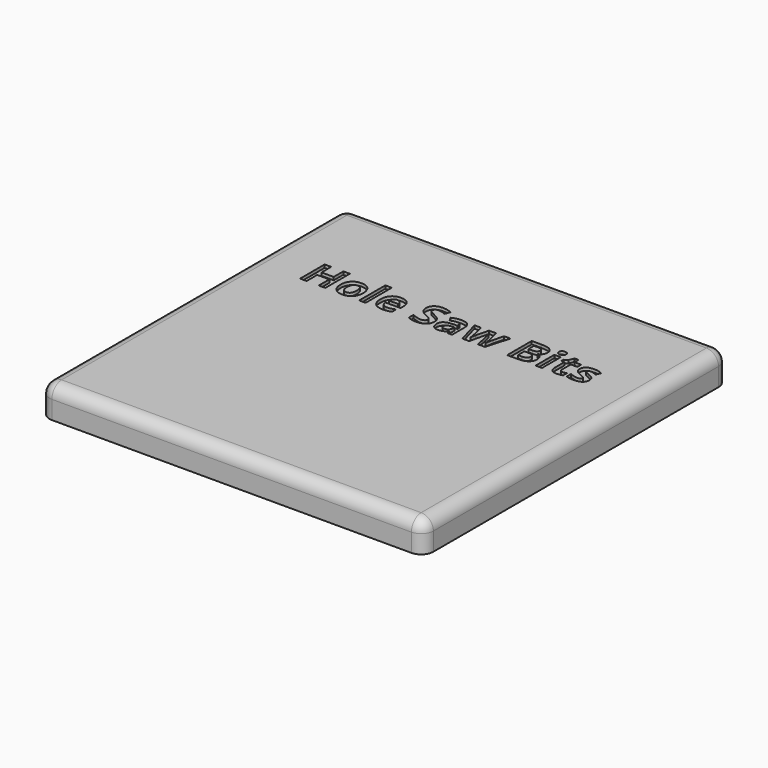
from build123d import *

# Parameters (mm, degrees)
F0_W         = 160.02
F0_H         = 158.75
F1_DEPTH     = 12.7
F2_R         = 5.08
F3_W         = 153.67
F3_H         = 153.67
F4_DEPTH     = 10.16
F6_TEXT_SIZE = 17.9435347854
F7_DEPTH     = 1.27


# Not quite as in the source:
# - Text() gives the source's letters only with a copy of the font that has no kerning and outlines rounded to 1/6400 em; it was checked with that copy


with BuildPart() as f1:
    # F0 (on Top) → F1 (new body)
    with BuildSketch(Plane.XY):
        Rectangle(F0_W, F0_H)
    extrude(amount=F1_DEPTH)

    # F2
    f2_edges = [f1.edges().sort_by_distance(p)[0] for p in [
        (80.01, 0, 12.7),
        (0, 79.375, 12.7),
        (-80.01, 0, 12.7),
        (0, -79.375, 12.7),
        (-80.01, 79.375, 6.35),
        (80.01, 79.375, 6.35),
        (80.01, -79.375, 6.35),
        (-80.01, -79.375, 6.35),
    ]]
    fillet(f2_edges, radius=F2_R)

    # F3 (on Top) → F4 (cut)
    with BuildSketch(Plane.XY):
        Rectangle(F3_W, F3_H)
    extrude(amount=F4_DEPTH, mode=Mode.SUBTRACT)

    # F6 (on offset) → F7 (cut)
    with BuildSketch(Plane.XY.offset(12.7)):
        with Locations((-60.5215802572, 29.9065754618)):
            Text('Hole Saw Bits', F6_TEXT_SIZE, font='Open Sans', font_style=FontStyle.BOLD, text_align=(TextAlign.LEFT, TextAlign.BOTTOM))
    extrude(amount=-F7_DEPTH, mode=Mode.SUBTRACT)


solid = f1.part
